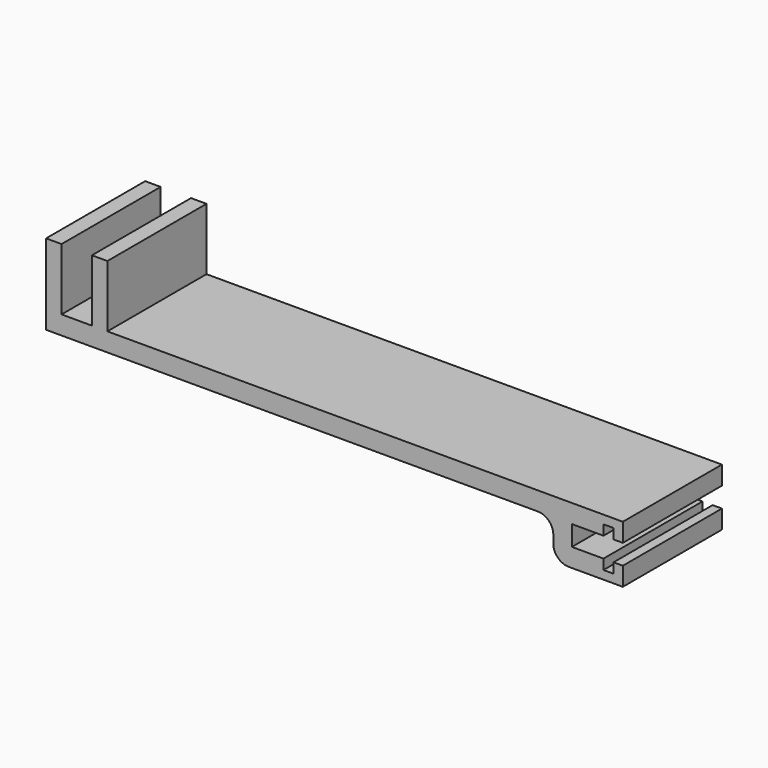
from build123d import *

# Parameters (mm, degrees)
F2_DEPTH     = 40
F3_TEXT_SIZE = 18.4504504505
F4_DEPTH     = 1


# Not quite as in the source:
# - Text() gives the source's letters only with a copy of the font that has no kerning and outlines rounded to 1/6400 em; it was checked with that copy


with BuildPart() as f2:
    # F1 (on Front) → F2 (new body)
    with BuildSketch(Plane.XZ):
        with BuildLine():
            Line((-186.25, 38.5), (-186.25, 12.5))
            Line((-186.25, 12.5), (-27.45, 12.5))
            ThreePointArc((-27.45, 12.5), (-23.9144660941, 11.0355339059), (-22.45, 7.5))
            Line((-22.45, 7.5), (-22.45, 5))
            ThreePointArc((-22.45, 5), (-20.9855339059, 1.4644660941), (-17.45, 0))
            Line((-17.45, 0), (0, 0))
            Line((0, 0), (0, 6))
            Line((0, 6), (-3, 6))
            Line((-3, 6), (-3, 2.75))
            Line((-3, 2.75), (-6.25, 2.75))
            Line((-6.25, 2.75), (-6.25, 6))
            Line((-6.25, 6), (-16.45, 6))
            Line((-16.45, 6), (-16.45, 12.5))
            Line((-16.45, 12.5), (-6.25, 12.5))
            Line((-6.25, 12.5), (-6.25, 15.75))
            Line((-6.25, 15.75), (-3, 15.75))
            Line((-3, 15.75), (-3, 12.5))
            Line((-3, 12.5), (0, 12.5))
            Line((0, 12.5), (0, 18.5))
            Line((0, 18.5), (-166.45, 18.5))
            Line((-166.45, 18.5), (-166.45, 38.5))
            Line((-166.45, 38.5), (-171.45, 38.5))
            Line((-171.45, 38.5), (-171.45, 18.5))
            Line((-171.45, 18.5), (-181.25, 18.5))
            Line((-181.25, 18.5), (-181.25, 38.5))
            Line((-181.25, 38.5), (-186.25, 38.5))
        make_face()
    extrude(amount=F2_DEPTH)

    # F3 (on face) → F4 (cut)
    with BuildSketch(Plane(origin=(-186.25, 0, 0), x_dir=(0, -1, 0), z_dir=(-1, 0, 0))):
        with Locations((0, 19.2156756757)):
            Text('HLM', F3_TEXT_SIZE, font='Open Sans', font_style=FontStyle.BOLDITALIC, text_align=(TextAlign.LEFT, TextAlign.BOTTOM))
    extrude(amount=-F4_DEPTH, mode=Mode.SUBTRACT)


solid = f2.part
